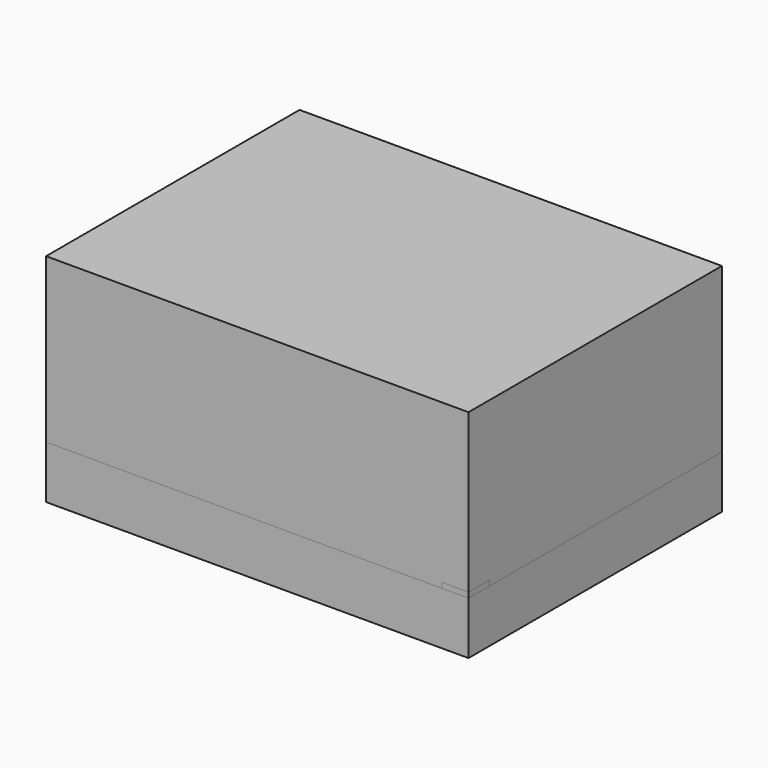
from build123d import *

# Parameters (mm, degrees)
F0_W     = 0.8
F0_H     = 0.6
F1_DEPTH = 0.1
F2_W     = 0.05
F2_H     = 0.05
F3_DEPTH = 0.01
F5_DEPTH = 0.01
F6_W     = 0.8
F6_H     = 0.6
F7_DEPTH = 0.3


with BuildPart() as f1:
    # F0 (on Top) → F1 (new body)
    with BuildSketch(Plane.XY):
        with Locations((-0.4, 0.3)):
            Rectangle(F0_W, F0_H)
    extrude(amount=F1_DEPTH)


with BuildPart() as f3:
    # F2 (on face) → F3 (new body)
    with BuildSketch(Plane.XY.offset(0.1)):
        with Locations((-0.025, 0.025)):
            Rectangle(F2_W, F2_H)
    extrude(amount=F3_DEPTH)


with BuildPart() as f5:
    # F4 (on face) → F5 (new body)
    with BuildSketch(Plane.XY.offset(0.1)):
        Polygon((0, 0.6), (-0.8, 0.6), (-0.8, 0), (-0.05, 0), (-0.05, 0.05), (0, 0.05), align=None)
    extrude(amount=F5_DEPTH)

    # F6 (on face) → F7 (join)
    with BuildSketch(Plane.XY.offset(0.11)):
        with Locations((-0.4, 0.3)):
            Rectangle(F6_W, F6_H)
    extrude(amount=F7_DEPTH)


solid = Compound([f1.part, f3.part, f5.part])
